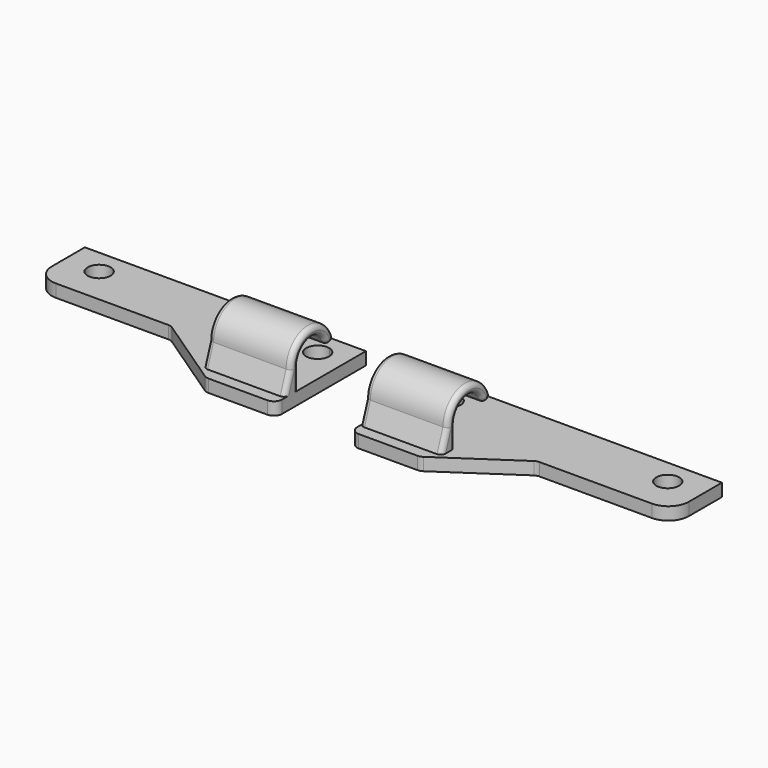
from build123d import *

# Parameters (mm, degrees)
F0_R      = 2.8
F1_DEPTH  = 3.1
F2_W      = 20
F2_H      = 2.3
F3_DEPTH  = 5.1
F3_FACE_W = 20
F3_FACE_H = 2.3
F5_ANGLE  = 170
F6_R      = 1.14999
F8_DEPTH  = 20
F9_R      = 1.14


# Not quite as in the source:
# - a fillet or chamfer is up to 0.001 mm smaller than in the source, because OpenCascade refuses the exact size
# - ends of sketch curves that miss each other by under 0.0002 mm in the source are joined


with BuildPart() as f1:
    # F0 (on Top) → F1 (new body)
    with BuildSketch(Plane.XY):
        with BuildLine():
            Line((37.938385576, 27.4999964178), (36.738385576, 27.4999964178))
            Line((36.738385576, 27.4999964178), (-20.7205781263, 27.4999964178))
            Line((-20.7205781263, 27.4999964178), (-25.7205781263, 27.4999966308))
            Line((-25.7205781263, 27.4999966308), (-25.7205781263, 22.4999966308))
            Line((-25.7205781263, 22.4999966308), (-25.7205781263, 17.3999966308))
            ThreePointArc((-25.7205781263, 17.3999966308), (-24.2561120322, 13.8644627249), (-20.7205781263, 12.3999966308))
            Line((-20.7205781263, 12.3999966308), (6.7794218737, 12.3999964178))
            ThreePointArc((6.7794218737, 12.3999964178), (7.3637845142, 12.312722301), (7.8971474214, 12.0585167222))
            Line((7.8971474214, 12.0585167222), (25.4316860469, 0.2414761133))
            ThreePointArc((25.4316860469, 0.2414761133), (25.9650489541, -0.0127294655), (26.5494115945, -0.1000035822))
            Line((26.5494115945, -0.1000035822), (40.938385576, -0.1000035822))
            ThreePointArc((40.938385576, -0.1000035822), (42.3525991384, 0.4857828554), (42.938385576, 1.8999964178))
            Line((42.938385576, 1.8999964178), (42.938385576, 12.3999964178))
            Line((42.938385576, 12.3999964178), (42.938385576, 22.4999964178))
            Line((42.938385576, 22.4999964178), (42.938385576, 27.4999964178))
            Line((42.938385576, 27.4999964178), (37.938385576, 27.4999964178))
        make_face()
        with Locations((-17.351614424, 21.3999971747)):
            Circle(F0_R, mode=Mode.SUBTRACT)
        with BuildLine():
            ThreePointArc((38.838385576, 21.3999964178), (33.8247912139, 19.6853535978), (36.738385576, 24.1110847601))
            ThreePointArc((36.738385576, 24.1110847601), (38.2519799381, 23.1146392377), (38.838385576, 21.3999964178))
        make_face(mode=Mode.SUBTRACT)
    extrude(amount=F1_DEPTH)

    # F2 (on face) → F3 (join)
    with BuildSketch(Plane.XY.offset(3.1)):
        with Locations((32.938385576, 5.6874617912)):
            Rectangle(F2_W, F2_H)
    extrude(amount=F3_DEPTH)

    # F3_face (on face) → F5 (revolve)
    with BuildSketch(Plane(origin=(32.938385576, 5.6874617912, 8.2), x_dir=(1, 0, 0), z_dir=(0, 0, 1))):
        Rectangle(F3_FACE_W, F3_FACE_H)
    revolve(axis=Axis((32.938385576, 11.2540264437, 8.2), (-1, 0, 0)), revolution_arc=F5_ANGLE)

    # F6 (radius 1.15 in the source; OpenCascade refuses exactly that, so slightly less here)
    f6_edges = [f1.edges().sort_by_distance(p)[0] for p in [
        (32.938386, 15.603494, 8.966928),
        (32.938386, 17.868551, 9.366319),
    ]]
    fillet(f6_edges, radius=F6_R)

    # F7 (on face) → F8 (join)
    with BuildSketch(Plane(origin=(22.938385576, 0, 0), x_dir=(0, -1, 0), z_dir=(-1, 0, 0))):
        Polygon((-2.7374617912, 3.1), (-4.5374617912, 8.2), (-4.5374617912, 3.1), align=None)
    extrude(amount=-F8_DEPTH)

    # F9
    f9_edges = [f1.edges().sort_by_distance(p)[0] for p in [
        (22.938386, 3.637462, 5.65),
        (22.938386, 9.976905, 14.794028),
        (42.938386, 3.637462, 5.65),
        (42.938386, 9.976905, 14.794028),
    ]]
    fillet(f9_edges, radius=F9_R)


with BuildPart() as f1_1:
    # F10: moved
    add(f1.part.moved(Location((-52.1, 0, 0))))


with BuildPart() as f11_1:
    # F11: instance of F1
    add(f1_1.part.mirror(Plane.YZ))


solid = Compound([f1_1.part, f11_1.part])
